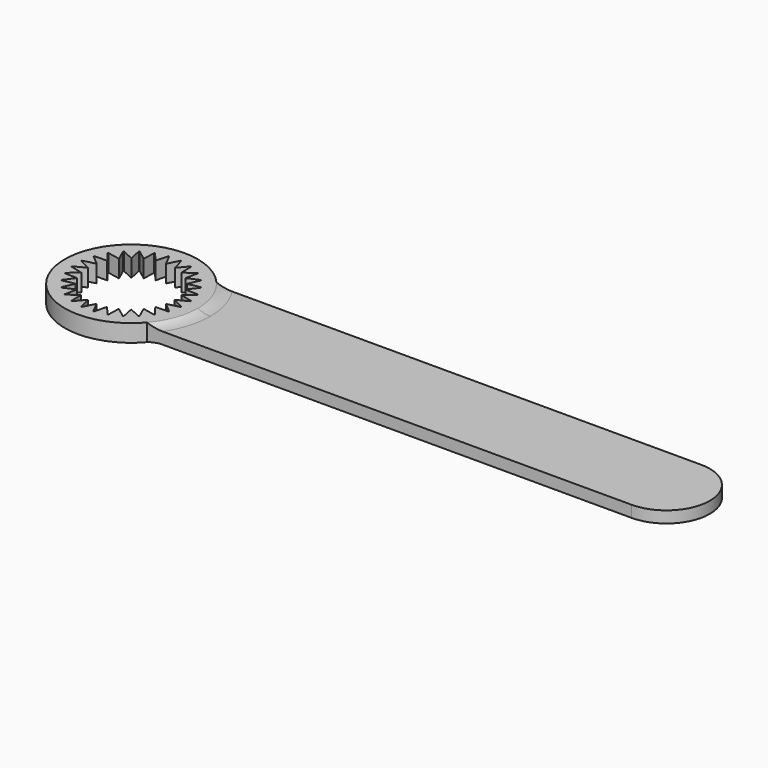
from build123d import *

# Parameters (mm, degrees)
F0_R         = 58.42
F0_R_2       = 48.26
F1_DEPTH     = 15.24
F4_DEPTH     = 5.08
F6_DEPTH     = 7.62
F7_T4_ANGLE  = 67.8542971522
F7_T9_ANGLE  = 67.8542971522
F7_T14_ANGLE = 67.8542971522
F7_T19_ANGLE = 67.8542971522


# Not quite as in the source:
# - a fillet or chamfer that OpenCascade refuses, or shapes differently, is made with other operations: its cross-section is extruded or revolved along the edge and cut away or added


with BuildPart() as f1:
    # F0 (on Top) → F1 (new body)
    with BuildSketch(Plane.XY):
        Circle(F0_R)
        Circle(F0_R_2, mode=Mode.SUBTRACT)
    extrude(amount=F1_DEPTH)

    # F3 (on offset) → F4 (join, symmetric)
    with BuildSketch(Plane.XY.offset(7.62)):
        with BuildLine():
            Line((469.9, 38.1), (44.2864132664, 38.1))
            ThreePointArc((44.2864132664, 38.1), (58.3891573479, 0), (44.2864132664, -38.1))
            Line((44.2864132664, -38.1), (469.9, -38.1))
            ThreePointArc((469.9, -38.1), (508, 0), (469.9, 38.1))
        make_face()
    extrude(amount=F4_DEPTH, both=True)

    # F5 (on offset) → F6 (join, symmetric)
    with BuildSketch(Plane.XY.offset(7.62)):
        with BuildLine():
            Line((-15.6318332701, 45.6582236691), (-8.4780475837, 37.1447534541))
            Line((-8.4780475837, 37.1447534541), (-5.7265656824, 47.9190363581))
            ThreePointArc((-5.7265656824, 47.9190363581), (-10.7388602727, 47.0500210419), (-15.6318332701, 45.6582236691))
        make_face()
        with BuildLine():
            Line((-5.08, 47.9918868143), (0, 38.1))
            Line((0, 38.1), (5.08, 47.9918868143))
            ThreePointArc((5.08, 47.9918868143), (0, 48.26), (-5.08, 47.9918868143))
        make_face()
        with BuildLine():
            Line((5.7265656824, 47.9190363581), (8.4780475837, 37.1447534541))
            Line((8.4780475837, 37.1447534541), (15.6318332701, 45.6582236691))
            ThreePointArc((15.6318332701, 45.6582236691), (10.7388602727, 47.0500210419), (5.7265656824, 47.9190363581))
        make_face()
        with BuildLine():
            Line((16.2459774494, 45.4433253263), (16.5309704604, 34.3269138671))
            Line((16.5309704604, 34.3269138671), (25.3998211473, 41.0350665369))
            ThreePointArc((25.3998211473, 41.0350665369), (20.9392292498, 43.480757565), (16.2459774494, 45.4433253263))
        make_face()
        with BuildLine():
            Line((25.9507480698, 40.6888962079), (23.7549614508, 29.787779482))
            Line((23.7549614508, 29.787779482), (33.8941559316, 34.354239821))
            ThreePointArc((33.8941559316, 34.354239821), (30.0896178377, 37.7311873439), (25.9507480698, 40.6888962079))
        make_face()
        with BuildLine():
            Line((34.354239821, 33.8941559316), (29.787779482, 23.7549614508))
            Line((29.787779482, 23.7549614508), (40.6888962079, 25.9507480698))
            ThreePointArc((40.6888962079, 25.9507480698), (37.7311873439, 30.0896178377), (34.354239821, 33.8941559316))
        make_face()
        with BuildLine():
            Line((41.0350665369, 25.3998211473), (34.3269138671, 16.5309704604))
            Line((34.3269138671, 16.5309704604), (45.4433253263, 16.2459774494))
            ThreePointArc((45.4433253263, 16.2459774494), (43.480757565, 20.9392292498), (41.0350665369, 25.3998211473))
        make_face()
        with BuildLine():
            Line((45.6582236691, 15.6318332701), (37.1447534541, 8.4780475837))
            Line((37.1447534541, 8.4780475837), (47.9190363581, 5.7265656824))
            ThreePointArc((47.9190363581, 5.7265656824), (47.0500210419, 10.7388602727), (45.6582236691, 15.6318332701))
        make_face()
        with BuildLine():
            Line((47.9918868143, 5.08), (38.1, 0))
            Line((38.1, 0), (47.9918868143, -5.08))
            ThreePointArc((47.9918868143, -5.08), (48.26, 0), (47.9918868143, 5.08))
        make_face()
        with BuildLine():
            Line((47.9190363581, -5.7265656824), (37.1447534541, -8.4780475837))
            Line((37.1447534541, -8.4780475837), (45.6582236691, -15.6318332701))
            ThreePointArc((45.6582236691, -15.6318332701), (47.0500210419, -10.7388602727), (47.9190363581, -5.7265656824))
        make_face()
        with BuildLine():
            Line((45.4433253263, -16.2459774494), (34.3269138671, -16.5309704604))
            Line((34.3269138671, -16.5309704604), (41.0350665369, -25.3998211473))
            ThreePointArc((41.0350665369, -25.3998211473), (43.480757565, -20.9392292498), (45.4433253263, -16.2459774494))
        make_face()
        with BuildLine():
            Line((40.6888962079, -25.9507480698), (29.787779482, -23.7549614508))
            Line((29.787779482, -23.7549614508), (34.354239821, -33.8941559316))
            ThreePointArc((34.354239821, -33.8941559316), (37.7311873439, -30.0896178377), (40.6888962079, -25.9507480698))
        make_face()
        with BuildLine():
            Line((25.3998211473, -41.0350665369), (16.5309704604, -34.3269138671))
            Line((16.5309704604, -34.3269138671), (16.2459774494, -45.4433253263))
            ThreePointArc((16.2459774494, -45.4433253263), (20.9392292498, -43.480757565), (25.3998211473, -41.0350665369))
        make_face()
        with BuildLine():
            Line((15.6318332701, -45.6582236691), (8.4780475837, -37.1447534541))
            Line((8.4780475837, -37.1447534541), (5.7265656824, -47.9190363581))
            ThreePointArc((5.7265656824, -47.9190363581), (10.7388602727, -47.0500210419), (15.6318332701, -45.6582236691))
        make_face()
        with BuildLine():
            Line((5.08, -47.9918868143), (0, -38.1))
            Line((0, -38.1), (-5.08, -47.9918868143))
            ThreePointArc((-5.08, -47.9918868143), (0, -48.26), (5.08, -47.9918868143))
        make_face()
        with BuildLine():
            Line((33.8941559316, -34.354239821), (23.7549614508, -29.787779482))
            Line((23.7549614508, -29.787779482), (25.9507480698, -40.6888962079))
            ThreePointArc((25.9507480698, -40.6888962079), (30.0896178377, -37.7311873439), (33.8941559316, -34.354239821))
        make_face()
        with BuildLine():
            Line((-5.7265656824, -47.9190363581), (-8.4780475837, -37.1447534541))
            Line((-8.4780475837, -37.1447534541), (-15.6318332701, -45.6582236691))
            ThreePointArc((-15.6318332701, -45.6582236691), (-10.7388602727, -47.0500210419), (-5.7265656824, -47.9190363581))
        make_face()
        with BuildLine():
            Line((-16.2459774494, -45.4433253263), (-16.5309704604, -34.3269138671))
            Line((-16.5309704604, -34.3269138671), (-25.3998211473, -41.0350665369))
            ThreePointArc((-25.3998211473, -41.0350665369), (-20.9392292498, -43.480757565), (-16.2459774494, -45.4433253263))
        make_face()
        with BuildLine():
            Line((-25.9507480698, -40.6888962079), (-23.7549614508, -29.787779482))
            Line((-23.7549614508, -29.787779482), (-33.8941559316, -34.354239821))
            ThreePointArc((-33.8941559316, -34.354239821), (-30.0896178377, -37.7311873439), (-25.9507480698, -40.6888962079))
        make_face()
        with BuildLine():
            Line((-34.354239821, -33.8941559316), (-29.787779482, -23.7549614508))
            Line((-29.787779482, -23.7549614508), (-40.6888962079, -25.9507480698))
            ThreePointArc((-40.6888962079, -25.9507480698), (-37.7311873439, -30.0896178377), (-34.354239821, -33.8941559316))
        make_face()
        with BuildLine():
            Line((-41.0350665369, -25.3998211473), (-34.3269138671, -16.5309704604))
            Line((-34.3269138671, -16.5309704604), (-45.4433253263, -16.2459774494))
            ThreePointArc((-45.4433253263, -16.2459774494), (-43.480757565, -20.9392292498), (-41.0350665369, -25.3998211473))
        make_face()
        with BuildLine():
            Line((-45.6582236691, -15.6318332701), (-37.1447534541, -8.4780475837))
            Line((-37.1447534541, -8.4780475837), (-47.9190363581, -5.7265656824))
            ThreePointArc((-47.9190363581, -5.7265656824), (-47.0500210419, -10.7388602727), (-45.6582236691, -15.6318332701))
        make_face()
        with BuildLine():
            Line((-47.9918868143, -5.08), (-38.1, 0))
            Line((-38.1, 0), (-47.9918868143, 5.08))
            ThreePointArc((-47.9918868143, 5.08), (-48.26, 0), (-47.9918868143, -5.08))
        make_face()
        with BuildLine():
            Line((-47.9190363581, 5.7265656824), (-37.1447534541, 8.4780475837))
            Line((-37.1447534541, 8.4780475837), (-45.6582236691, 15.6318332701))
            ThreePointArc((-45.6582236691, 15.6318332701), (-47.0500210419, 10.7388602727), (-47.9190363581, 5.7265656824))
        make_face()
        with BuildLine():
            Line((-45.4433253263, 16.2459774494), (-34.3269138671, 16.5309704604))
            Line((-34.3269138671, 16.5309704604), (-41.0350665369, 25.3998211473))
            ThreePointArc((-41.0350665369, 25.3998211473), (-43.480757565, 20.9392292498), (-45.4433253263, 16.2459774494))
        make_face()
        with BuildLine():
            Line((-40.6888962079, 25.9507480698), (-29.787779482, 23.7549614508))
            Line((-29.787779482, 23.7549614508), (-34.354239821, 33.8941559316))
            ThreePointArc((-34.354239821, 33.8941559316), (-37.7311873439, 30.0896178377), (-40.6888962079, 25.9507480698))
        make_face()
        with BuildLine():
            Line((-33.8941559316, 34.354239821), (-23.7549614508, 29.787779482))
            Line((-23.7549614508, 29.787779482), (-25.9507480698, 40.6888962079))
            ThreePointArc((-25.9507480698, 40.6888962079), (-30.0896178377, 37.7311873439), (-33.8941559316, 34.354239821))
        make_face()
        with BuildLine():
            Line((-25.3998211473, 41.0350665369), (-16.5309704604, 34.3269138671))
            Line((-16.5309704604, 34.3269138671), (-16.2459774494, 45.4433253263))
            ThreePointArc((-16.2459774494, 45.4433253263), (-20.9392292498, 43.480757565), (-25.3998211473, 41.0350665369))
        make_face()
    extrude(amount=F6_DEPTH, both=True)

    # F7: fillet of radius 25.4 on 4 edges, made by hand


with BuildPart() as f7_tool2:
    # F7_s3 → F7_t4 (revolve)
    with BuildSketch(Plane.XZ):
        with BuildLine():
            ThreePointArc((58.42, 15.24), (63.8119906537, 13.3431423642), (69.4916033166, 12.7))
            Line((69.4916033166, 12.7), (58.42, 12.7))
            Line((58.42, 12.7), (58.42, 15.24))
        make_face()
    revolve(axis=Axis((0, 0, 12.7), (0, 0, -1)), revolution_arc=F7_T4_ANGLE)

    split(bisect_by=Plane.XZ.offset(38.1), keep=Keep.BOTTOM)


with BuildPart() as f1_1:
    add(f1.part)

    # F7_t1: union F7_tool2
    add(f7_tool2.part)


with BuildPart() as f7_tool7:
    # F7_s8 → F7_t9 (revolve)
    with BuildSketch(Plane(origin=(0, 0, 0), x_dir=(0, 0, 1), z_dir=(-0.9262282352, 0.376963203, 0))):
        with BuildLine():
            ThreePointArc((15.24, 58.42), (13.3431423642, 63.8119906537), (12.7, 69.4916033166))
            Line((12.7, 69.4916033166), (12.7, 58.42))
            Line((12.7, 58.42), (15.24, 58.42))
        make_face()
    revolve(axis=Axis((0, 0, 12.7), (0, 0, -1)), revolution_arc=F7_T9_ANGLE)

    split(bisect_by=Plane.XZ.offset(-38.1), keep=Keep.TOP)


with BuildPart() as f1_2:
    add(f1_1.part)

    # F7_t6: union F7_tool7
    add(f7_tool7.part)


with BuildPart() as f7_tool12:
    # F7_s13 → F7_t14 (revolve)
    with BuildSketch(Plane.XZ):
        with BuildLine():
            ThreePointArc((58.42, 0), (63.8119906537, 1.8968576358), (69.4916033166, 2.54))
            Line((69.4916033166, 2.54), (58.42, 2.54))
            Line((58.42, 2.54), (58.42, 0))
        make_face()
    revolve(axis=Axis((0, 0, 2.54), (0, 0, -1)), revolution_arc=F7_T14_ANGLE)

    split(bisect_by=Plane.XZ.offset(38.1), keep=Keep.BOTTOM)


with BuildPart() as f1_3:
    add(f1_2.part)

    # F7_t11: union F7_tool12
    add(f7_tool12.part)


with BuildPart() as f7_tool17:
    # F7_s18 → F7_t19 (revolve)
    with BuildSketch(Plane(origin=(0, 0, 0), x_dir=(0, 0, 1), z_dir=(-0.9262282352, 0.376963203, 0))):
        with BuildLine():
            ThreePointArc((0, 58.42), (1.8968576358, 63.8119906537), (2.54, 69.4916033166))
            Line((2.54, 69.4916033166), (2.54, 58.42))
            Line((2.54, 58.42), (0, 58.42))
        make_face()
    revolve(axis=Axis((0, 0, 2.54), (0, 0, -1)), revolution_arc=F7_T19_ANGLE)

    split(bisect_by=Plane.XZ.offset(-38.1), keep=Keep.TOP)


with BuildPart() as f1_4:
    add(f1_3.part)

    # F7_t16: union F7_tool17
    add(f7_tool17.part)


solid = f1_4.part
